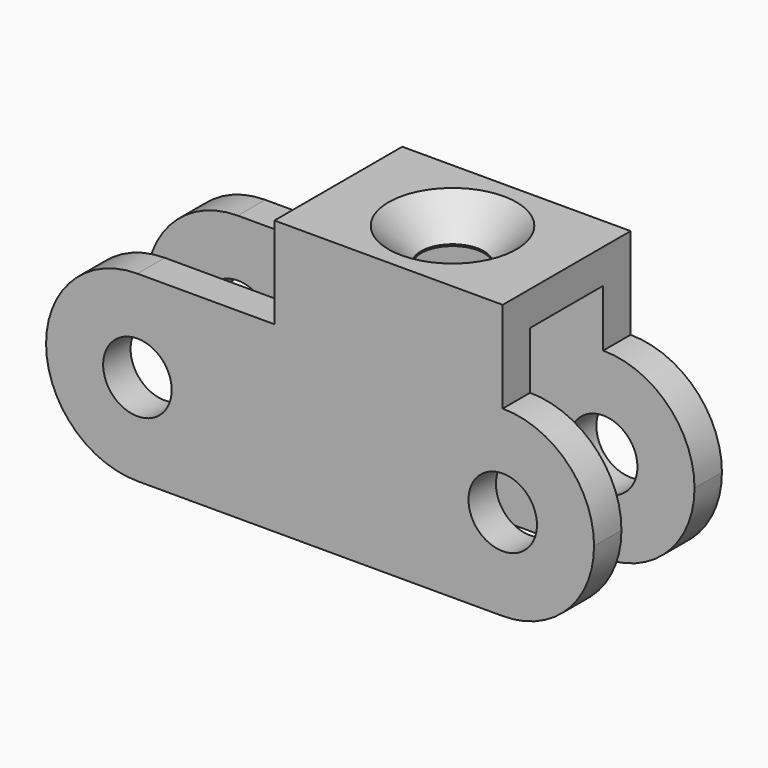
from build123d import *

# Parameters (mm, degrees)
F0_R           = 3
F0_W           = 20
F0_H           = 8
F1_DEPTH       = 14
F2_R           = 7.99999
F3_W           = 62.9811411479
F3_H           = 8
F4_DEPTH       = 21
F6_D           = 5.5
F6_CSINK_D     = 11.2
F6_CSINK_ANGLE = 90


# Not quite as in the source:
# - a fillet or chamfer is up to 0.001 mm smaller than in the source, because OpenCascade refuses the exact size


with BuildPart() as f1:
    # F0 (on Front) → F1 (new body)
    with BuildSketch(Plane.XZ):
        Polygon((0, 16), (0, 0), (48, 0), (48, 16), (40, 16), (20, 16), align=None)
        with Locations((8, 8)):
            Circle(F0_R, mode=Mode.SUBTRACT)
        with Locations((40, 8)):
            Circle(F0_R, mode=Mode.SUBTRACT)
        with Locations((30, 20)):
            Rectangle(F0_W, F0_H)
    extrude(amount=F1_DEPTH)

    # F2 (radius 8 in the source; OpenCascade refuses exactly that, so slightly less here)
    f2_edges = [f1.edges().sort_by_distance(p)[0] for p in [
        (0, -7, 16),
        (0, -7, 0),
        (48, -7, 16),
        (48, -7, 0),
    ]]
    fillet(f2_edges, radius=F2_R)

    # F3 (on face) → F4 (cut)
    with BuildSketch(Plane(origin=(0, 0, 0), x_dir=(1, 0, 0), z_dir=(0, 0, -1))):
        with Locations((30.1177082001, 7)):
            Rectangle(F3_W, F3_H)
    extrude(amount=-F4_DEPTH, mode=Mode.SUBTRACT)

    # F6 (through all)
    with Locations(Plane.XY.offset(24)):
        with Locations((30, -7)):
            CounterSinkHole(F6_D / 2, F6_CSINK_D / 2, counter_sink_angle=F6_CSINK_ANGLE)


solid = f1.part
